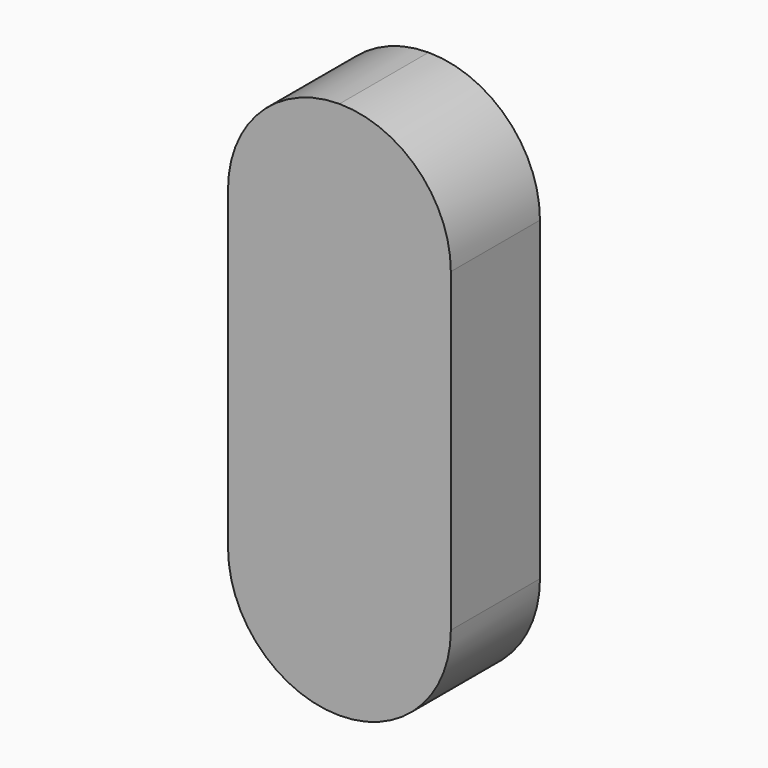
from build123d import *

# Parameters (mm, degrees)
F0_W     = 60
F0_H     = 145
F1_DEPTH = 30
F2_R     = 29.99999


# Not quite as in the source:
# - a fillet or chamfer is up to 0.001 mm smaller than in the source, because OpenCascade refuses the exact size


with BuildPart() as f1:
    # F0 (on Front) → F1 (new body)
    with BuildSketch(Plane.XZ):
        with Locations((30, 72.5)):
            Rectangle(F0_W, F0_H)
    extrude(amount=F1_DEPTH)

    # F2 (radius 30 in the source; OpenCascade refuses exactly that, so slightly less here)
    f2_edges = [f1.edges().sort_by_distance(p)[0] for p in [
        (0, -15, 145),
        (60, -15, 145),
        (0, -15, 0),
        (60, -15, 0),
    ]]
    fillet(f2_edges, radius=F2_R)


solid = f1.part
